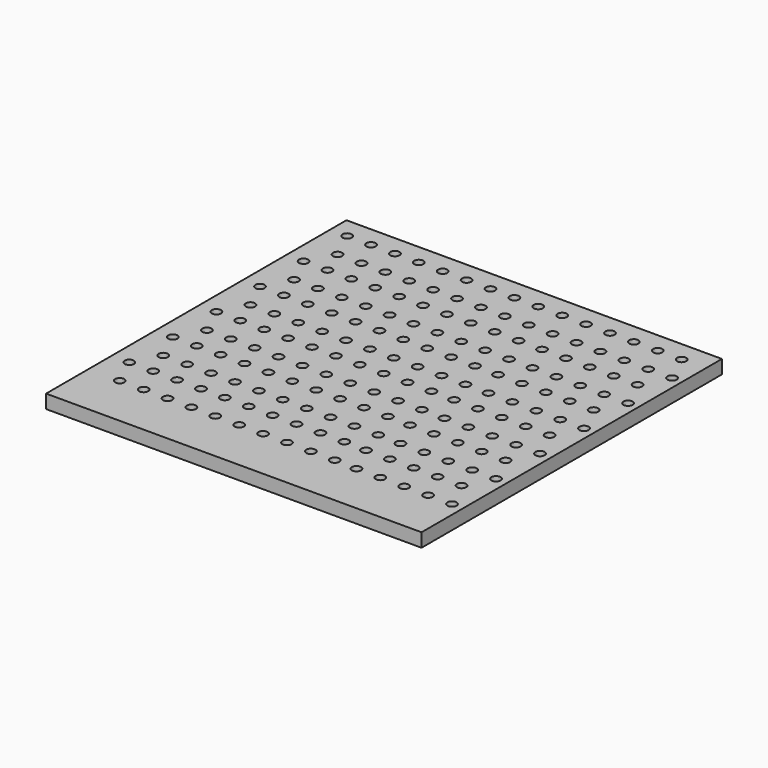
from build123d import *

# Parameters (mm, degrees)
F0_W     = 110
F0_H     = 110
F0_R     = 1.35
F1_DEPTH = 4


# Not quite as in the source:
# - a feature names something its author has since deleted; it is built from what else it names


with BuildPart() as f1:
    # F0 (on Top) → F1 (new body)
    with BuildSketch(Plane.XY):
        with Locations((-18.9387425125, -57.1583950296)):
            Rectangle(F0_W, F0_H)
        with Locations((-64.7594391714, -96.6581940938)):
            Circle(F0_R, mode=Mode.SUBTRACT)
        with Locations((-68.7594391714, -88.1581940938)):
            Circle(F0_R, mode=Mode.SUBTRACT)
        with Locations((-61.7594391714, -88.1581940938)):
            Circle(F0_R, mode=Mode.SUBTRACT)
        with Locations((-57.7594391714, -96.6581940938)):
            Circle(F0_R, mode=Mode.SUBTRACT)
        with Locations((-50.7594391714, -96.6581940938)):
            Circle(F0_R, mode=Mode.SUBTRACT)
        with Locations((-54.7594391714, -88.1581940938)):
            Circle(F0_R, mode=Mode.SUBTRACT)
        with Locations((-47.7594391714, -88.1581940938)):
            Circle(F0_R, mode=Mode.SUBTRACT)
        with Locations((-43.7594391714, -96.6581940938)):
            Circle(F0_R, mode=Mode.SUBTRACT)
        with Locations((-36.7594391714, -96.6581940938)):
            Circle(F0_R, mode=Mode.SUBTRACT)
        with Locations((-40.7594391714, -88.1581940938)):
            Circle(F0_R, mode=Mode.SUBTRACT)
        with Locations((-33.7594391714, -88.1581940938)):
            Circle(F0_R, mode=Mode.SUBTRACT)
        with Locations((-29.7594391714, -96.6581940938)):
            Circle(F0_R, mode=Mode.SUBTRACT)
        with Locations((-22.7594391714, -96.6581940938)):
            Circle(F0_R, mode=Mode.SUBTRACT)
        with Locations((-26.7594391714, -88.1581940938)):
            Circle(F0_R, mode=Mode.SUBTRACT)
        with Locations((-19.7594391714, -88.1581940938)):
            Circle(F0_R, mode=Mode.SUBTRACT)
        with Locations((-64.7952998396, -80.658234281)):
            Circle(F0_R, mode=Mode.SUBTRACT)
        with Locations((-68.7952998396, -72.158234281)):
            Circle(F0_R, mode=Mode.SUBTRACT)
        with Locations((-61.7952998396, -72.158234281)):
            Circle(F0_R, mode=Mode.SUBTRACT)
        with Locations((-57.7952998396, -80.658234281)):
            Circle(F0_R, mode=Mode.SUBTRACT)
        with Locations((-50.7952998396, -80.658234281)):
            Circle(F0_R, mode=Mode.SUBTRACT)
        with Locations((-54.7952998396, -72.158234281)):
            Circle(F0_R, mode=Mode.SUBTRACT)
        with Locations((-47.7952998396, -72.158234281)):
            Circle(F0_R, mode=Mode.SUBTRACT)
        with Locations((-64.8311605078, -64.6582744682)):
            Circle(F0_R, mode=Mode.SUBTRACT)
        with Locations((-57.8311605078, -64.6582744682)):
            Circle(F0_R, mode=Mode.SUBTRACT)
        with Locations((-50.8311605078, -64.6582744682)):
            Circle(F0_R, mode=Mode.SUBTRACT)
        with Locations((-43.7952998396, -80.658234281)):
            Circle(F0_R, mode=Mode.SUBTRACT)
        with Locations((-36.7952998396, -80.658234281)):
            Circle(F0_R, mode=Mode.SUBTRACT)
        with Locations((-40.7952998396, -72.158234281)):
            Circle(F0_R, mode=Mode.SUBTRACT)
        with Locations((-33.7952998396, -72.158234281)):
            Circle(F0_R, mode=Mode.SUBTRACT)
        with Locations((-29.7952998396, -80.658234281)):
            Circle(F0_R, mode=Mode.SUBTRACT)
        with Locations((-22.7952998396, -80.658234281)):
            Circle(F0_R, mode=Mode.SUBTRACT)
        with Locations((-26.7952998396, -72.158234281)):
            Circle(F0_R, mode=Mode.SUBTRACT)
        with Locations((-19.7952998396, -72.158234281)):
            Circle(F0_R, mode=Mode.SUBTRACT)
        with Locations((-43.8311605078, -64.6582744682)):
            Circle(F0_R, mode=Mode.SUBTRACT)
        with Locations((-36.8311605078, -64.6582744682)):
            Circle(F0_R, mode=Mode.SUBTRACT)
        with Locations((-29.8311605078, -64.6582744682)):
            Circle(F0_R, mode=Mode.SUBTRACT)
        with Locations((-22.8311605078, -64.6582744682)):
            Circle(F0_R, mode=Mode.SUBTRACT)
        with Locations((-15.7594391714, -96.6581940938)):
            Circle(F0_R, mode=Mode.SUBTRACT)
        with Locations((-8.7594391714, -96.6581940938)):
            Circle(F0_R, mode=Mode.SUBTRACT)
        with Locations((-12.7594391714, -88.1581940938)):
            Circle(F0_R, mode=Mode.SUBTRACT)
        with Locations((-5.7594391714, -88.1581940938)):
            Circle(F0_R, mode=Mode.SUBTRACT)
        with Locations((-1.7594391714, -96.6581940938)):
            Circle(F0_R, mode=Mode.SUBTRACT)
        with Locations((4.7549700499, -96.8664198815)):
            Circle(F0_R, mode=Mode.SUBTRACT)
        with Locations((0.7549700499, -88.3664198815)):
            Circle(F0_R, mode=Mode.SUBTRACT)
        with Locations((7.7549700499, -88.3664198815)):
            Circle(F0_R, mode=Mode.SUBTRACT)
        with Locations((11.7549700499, -96.8664198815)):
            Circle(F0_R, mode=Mode.SUBTRACT)
        with Locations((18.7549700499, -96.8664198815)):
            Circle(F0_R, mode=Mode.SUBTRACT)
        with Locations((14.7549700499, -88.3664198815)):
            Circle(F0_R, mode=Mode.SUBTRACT)
        with Locations((21.7549700499, -88.3664198815)):
            Circle(F0_R, mode=Mode.SUBTRACT)
        with Locations((25.7549700499, -96.8664198815)):
            Circle(F0_R, mode=Mode.SUBTRACT)
        with Locations((32.7549700499, -96.8664198815)):
            Circle(F0_R, mode=Mode.SUBTRACT)
        with Locations((28.7549700499, -88.3664198815)):
            Circle(F0_R, mode=Mode.SUBTRACT)
        with Locations((-15.7952998396, -80.658234281)):
            Circle(F0_R, mode=Mode.SUBTRACT)
        with Locations((-8.7952998396, -80.658234281)):
            Circle(F0_R, mode=Mode.SUBTRACT)
        with Locations((-12.7952998396, -72.158234281)):
            Circle(F0_R, mode=Mode.SUBTRACT)
        with Locations((-5.7952998396, -72.158234281)):
            Circle(F0_R, mode=Mode.SUBTRACT)
        with Locations((-1.7952998396, -80.658234281)):
            Circle(F0_R, mode=Mode.SUBTRACT)
        with Locations((4.8162275374, -80.8248149111)):
            Circle(F0_R, mode=Mode.SUBTRACT)
        with Locations((0.8162275374, -72.3248149111)):
            Circle(F0_R, mode=Mode.SUBTRACT)
        with Locations((7.8162275374, -72.3248149111)):
            Circle(F0_R, mode=Mode.SUBTRACT)
        with Locations((-15.8311605078, -64.6582744682)):
            Circle(F0_R, mode=Mode.SUBTRACT)
        with Locations((-8.8311605078, -64.6582744682)):
            Circle(F0_R, mode=Mode.SUBTRACT)
        with Locations((-1.8311605078, -64.6582744682)):
            Circle(F0_R, mode=Mode.SUBTRACT)
        with Locations((4.877485025, -64.7832099407)):
            Circle(F0_R, mode=Mode.SUBTRACT)
        with Locations((11.8162275374, -80.8248149111)):
            Circle(F0_R, mode=Mode.SUBTRACT)
        with Locations((18.8162275374, -80.8248149111)):
            Circle(F0_R, mode=Mode.SUBTRACT)
        with Locations((14.8162275374, -72.3248149111)):
            Circle(F0_R, mode=Mode.SUBTRACT)
        with Locations((21.8162275374, -72.3248149111)):
            Circle(F0_R, mode=Mode.SUBTRACT)
        with Locations((25.8162275374, -80.8248149111)):
            Circle(F0_R, mode=Mode.SUBTRACT)
        with Locations((32.8162275374, -80.8248149111)):
            Circle(F0_R, mode=Mode.SUBTRACT)
        with Locations((28.8162275374, -72.3248149111)):
            Circle(F0_R, mode=Mode.SUBTRACT)
        with Locations((11.877485025, -64.7832099407)):
            Circle(F0_R, mode=Mode.SUBTRACT)
        with Locations((18.877485025, -64.7832099407)):
            Circle(F0_R, mode=Mode.SUBTRACT)
        with Locations((25.877485025, -64.7832099407)):
            Circle(F0_R, mode=Mode.SUBTRACT)
        with Locations((32.877485025, -64.7832099407)):
            Circle(F0_R, mode=Mode.SUBTRACT)
        with Locations((-68.8311605078, -56.1582744682)):
            Circle(F0_R, mode=Mode.SUBTRACT)
        with Locations((-61.8311605078, -56.1582744682)):
            Circle(F0_R, mode=Mode.SUBTRACT)
        with Locations((-64.8670211761, -48.6583146553)):
            Circle(F0_R, mode=Mode.SUBTRACT)
        with Locations((-54.8311605078, -56.1582744682)):
            Circle(F0_R, mode=Mode.SUBTRACT)
        with Locations((-47.8311605078, -56.1582744682)):
            Circle(F0_R, mode=Mode.SUBTRACT)
        with Locations((-57.8670211761, -48.6583146553)):
            Circle(F0_R, mode=Mode.SUBTRACT)
        with Locations((-50.8670211761, -48.6583146553)):
            Circle(F0_R, mode=Mode.SUBTRACT)
        with Locations((-68.8670211761, -40.1583146553)):
            Circle(F0_R, mode=Mode.SUBTRACT)
        with Locations((-61.8670211761, -40.1583146553)):
            Circle(F0_R, mode=Mode.SUBTRACT)
        with Locations((-64.9028818443, -32.6583548425)):
            Circle(F0_R, mode=Mode.SUBTRACT)
        with Locations((-54.8670211761, -40.1583146553)):
            Circle(F0_R, mode=Mode.SUBTRACT)
        with Locations((-47.8670211761, -40.1583146553)):
            Circle(F0_R, mode=Mode.SUBTRACT)
        with Locations((-57.9028818443, -32.6583548425)):
            Circle(F0_R, mode=Mode.SUBTRACT)
        with Locations((-50.9028818443, -32.6583548425)):
            Circle(F0_R, mode=Mode.SUBTRACT)
        with Locations((-40.8311605078, -56.1582744682)):
            Circle(F0_R, mode=Mode.SUBTRACT)
        with Locations((-33.8311605078, -56.1582744682)):
            Circle(F0_R, mode=Mode.SUBTRACT)
        with Locations((-43.8670211761, -48.6583146553)):
            Circle(F0_R, mode=Mode.SUBTRACT)
        with Locations((-36.8670211761, -48.6583146553)):
            Circle(F0_R, mode=Mode.SUBTRACT)
        with Locations((-26.8311605078, -56.1582744682)):
            Circle(F0_R, mode=Mode.SUBTRACT)
        with Locations((-19.8311605078, -56.1582744682)):
            Circle(F0_R, mode=Mode.SUBTRACT)
        with Locations((-29.8670211761, -48.6583146553)):
            Circle(F0_R, mode=Mode.SUBTRACT)
        with Locations((-22.8670211761, -48.6583146553)):
            Circle(F0_R, mode=Mode.SUBTRACT)
        with Locations((-40.8670211761, -40.1583146553)):
            Circle(F0_R, mode=Mode.SUBTRACT)
        with Locations((-33.8670211761, -40.1583146553)):
            Circle(F0_R, mode=Mode.SUBTRACT)
        with Locations((-43.9028818443, -32.6583548425)):
            Circle(F0_R, mode=Mode.SUBTRACT)
        with Locations((-36.9028818443, -32.6583548425)):
            Circle(F0_R, mode=Mode.SUBTRACT)
        with Locations((-26.8670211761, -40.1583146553)):
            Circle(F0_R, mode=Mode.SUBTRACT)
        with Locations((-19.8670211761, -40.1583146553)):
            Circle(F0_R, mode=Mode.SUBTRACT)
        with Locations((-29.9028818443, -32.6583548425)):
            Circle(F0_R, mode=Mode.SUBTRACT)
        with Locations((-22.9028818443, -32.6583548425)):
            Circle(F0_R, mode=Mode.SUBTRACT)
        with Locations((-68.9028818443, -24.1583548425)):
            Circle(F0_R, mode=Mode.SUBTRACT)
        with Locations((-61.9028818443, -24.1583548425)):
            Circle(F0_R, mode=Mode.SUBTRACT)
        with Locations((-64.9387425125, -16.6583950296)):
            Circle(F0_R, mode=Mode.SUBTRACT)
        with Locations((-54.9028818443, -24.1583548425)):
            Circle(F0_R, mode=Mode.SUBTRACT)
        with Locations((-47.9028818443, -24.1583548425)):
            Circle(F0_R, mode=Mode.SUBTRACT)
        with Locations((-57.9387425125, -16.6583950296)):
            Circle(F0_R, mode=Mode.SUBTRACT)
        with Locations((-50.9387425125, -16.6583950296)):
            Circle(F0_R, mode=Mode.SUBTRACT)
        with Locations((-68.9387425125, -8.1583950296)):
            Circle(F0_R, mode=Mode.SUBTRACT)
        with Locations((-61.9387425125, -8.1583950296)):
            Circle(F0_R, mode=Mode.SUBTRACT)
        with Locations((-54.9387425125, -8.1583950296)):
            Circle(F0_R, mode=Mode.SUBTRACT)
        with Locations((-47.9387425125, -8.1583950296)):
            Circle(F0_R, mode=Mode.SUBTRACT)
        with Locations((-40.9028818443, -24.1583548425)):
            Circle(F0_R, mode=Mode.SUBTRACT)
        with Locations((-33.9028818443, -24.1583548425)):
            Circle(F0_R, mode=Mode.SUBTRACT)
        with Locations((-43.9387425125, -16.6583950296)):
            Circle(F0_R, mode=Mode.SUBTRACT)
        with Locations((-36.9387425125, -16.6583950296)):
            Circle(F0_R, mode=Mode.SUBTRACT)
        with Locations((-26.9028818443, -24.1583548425)):
            Circle(F0_R, mode=Mode.SUBTRACT)
        with Locations((-19.9028818443, -24.1583548425)):
            Circle(F0_R, mode=Mode.SUBTRACT)
        with Locations((-29.9387425125, -16.6583950296)):
            Circle(F0_R, mode=Mode.SUBTRACT)
        with Locations((-22.9387425125, -16.6583950296)):
            Circle(F0_R, mode=Mode.SUBTRACT)
        with Locations((-40.9387425125, -8.1583950296)):
            Circle(F0_R, mode=Mode.SUBTRACT)
        with Locations((-33.9387425125, -8.1583950296)):
            Circle(F0_R, mode=Mode.SUBTRACT)
        with Locations((-26.9387425125, -8.1583950296)):
            Circle(F0_R, mode=Mode.SUBTRACT)
        with Locations((-19.9387425125, -8.1583950296)):
            Circle(F0_R, mode=Mode.SUBTRACT)
        with Locations((-12.8311605078, -56.1582744682)):
            Circle(F0_R, mode=Mode.SUBTRACT)
        with Locations((-5.8311605078, -56.1582744682)):
            Circle(F0_R, mode=Mode.SUBTRACT)
        with Locations((-15.8670211761, -48.6583146553)):
            Circle(F0_R, mode=Mode.SUBTRACT)
        with Locations((-8.8670211761, -48.6583146553)):
            Circle(F0_R, mode=Mode.SUBTRACT)
        with Locations((0.877485025, -56.2832099407)):
            Circle(F0_R, mode=Mode.SUBTRACT)
        with Locations((7.877485025, -56.2832099407)):
            Circle(F0_R, mode=Mode.SUBTRACT)
        with Locations((-1.8670211761, -48.6583146553)):
            Circle(F0_R, mode=Mode.SUBTRACT)
        with Locations((4.9387425125, -48.7416049704)):
            Circle(F0_R, mode=Mode.SUBTRACT)
        with Locations((-12.8670211761, -40.1583146553)):
            Circle(F0_R, mode=Mode.SUBTRACT)
        with Locations((-5.8670211761, -40.1583146553)):
            Circle(F0_R, mode=Mode.SUBTRACT)
        with Locations((-15.9028818443, -32.6583548425)):
            Circle(F0_R, mode=Mode.SUBTRACT)
        with Locations((-8.9028818443, -32.6583548425)):
            Circle(F0_R, mode=Mode.SUBTRACT)
        with Locations((0.9387425125, -40.2416049704)):
            Circle(F0_R, mode=Mode.SUBTRACT)
        with Locations((7.9387425125, -40.2416049704)):
            Circle(F0_R, mode=Mode.SUBTRACT)
        with Locations((-1.9028818443, -32.6583548425)):
            Circle(F0_R, mode=Mode.SUBTRACT)
        with Locations((5, -32.7)):
            Circle(F0_R, mode=Mode.SUBTRACT)
        with Locations((14.877485025, -56.2832099407)):
            Circle(F0_R, mode=Mode.SUBTRACT)
        with Locations((21.877485025, -56.2832099407)):
            Circle(F0_R, mode=Mode.SUBTRACT)
        with Locations((11.9387425125, -48.7416049704)):
            Circle(F0_R, mode=Mode.SUBTRACT)
        with Locations((18.9387425125, -48.7416049704)):
            Circle(F0_R, mode=Mode.SUBTRACT)
        with Locations((28.877485025, -56.2832099407)):
            Circle(F0_R, mode=Mode.SUBTRACT)
        with Locations((25.9387425125, -48.7416049704)):
            Circle(F0_R, mode=Mode.SUBTRACT)
        with Locations((32.9387425125, -48.7416049704)):
            Circle(F0_R, mode=Mode.SUBTRACT)
        with Locations((14.9387425125, -40.2416049704)):
            Circle(F0_R, mode=Mode.SUBTRACT)
        with Locations((21.9387425125, -40.2416049704)):
            Circle(F0_R, mode=Mode.SUBTRACT)
        with Locations((12, -32.7)):
            Circle(F0_R, mode=Mode.SUBTRACT)
        with Locations((19, -32.7)):
            Circle(F0_R, mode=Mode.SUBTRACT)
        with Locations((28.9387425125, -40.2416049704)):
            Circle(F0_R, mode=Mode.SUBTRACT)
        with Locations((26, -32.7)):
            Circle(F0_R, mode=Mode.SUBTRACT)
        with Locations((33, -32.7)):
            Circle(F0_R, mode=Mode.SUBTRACT)
        with Locations((-12.9028818443, -24.1583548425)):
            Circle(F0_R, mode=Mode.SUBTRACT)
        with Locations((-5.9028818443, -24.1583548425)):
            Circle(F0_R, mode=Mode.SUBTRACT)
        with Locations((-15.9387425125, -16.6583950296)):
            Circle(F0_R, mode=Mode.SUBTRACT)
        with Locations((-8.9387425125, -16.6583950296)):
            Circle(F0_R, mode=Mode.SUBTRACT)
        with Locations((1, -24.2)):
            Circle(F0_R, mode=Mode.SUBTRACT)
        with Locations((8, -24.2)):
            Circle(F0_R, mode=Mode.SUBTRACT)
        with Locations((-1.9387425125, -16.6583950296)):
            Circle(F0_R, mode=Mode.SUBTRACT)
        with Locations((5.0612574875, -16.6583950296)):
            Circle(F0_R, mode=Mode.SUBTRACT)
        with Locations((-12.9387425125, -8.1583950296)):
            Circle(F0_R, mode=Mode.SUBTRACT)
        with Locations((-5.9387425125, -8.1583950296)):
            Circle(F0_R, mode=Mode.SUBTRACT)
        with Locations((1.0612574875, -8.1583950296)):
            Circle(F0_R, mode=Mode.SUBTRACT)
        with Locations((8.0612574875, -8.1583950296)):
            Circle(F0_R, mode=Mode.SUBTRACT)
        with Locations((15, -24.2)):
            Circle(F0_R, mode=Mode.SUBTRACT)
        with Locations((22, -24.2)):
            Circle(F0_R, mode=Mode.SUBTRACT)
        with Locations((12.0612574875, -16.6583950296)):
            Circle(F0_R, mode=Mode.SUBTRACT)
        with Locations((19.0612574875, -16.6583950296)):
            Circle(F0_R, mode=Mode.SUBTRACT)
        with Locations((29, -24.2)):
            Circle(F0_R, mode=Mode.SUBTRACT)
        with Locations((26.0612574875, -16.6583950296)):
            Circle(F0_R, mode=Mode.SUBTRACT)
        with Locations((33.0612574875, -16.6583950296)):
            Circle(F0_R, mode=Mode.SUBTRACT)
        with Locations((15.0612574875, -8.1583950296)):
            Circle(F0_R, mode=Mode.SUBTRACT)
        with Locations((22.0612574875, -8.1583950296)):
            Circle(F0_R, mode=Mode.SUBTRACT)
        with Locations((29.0612574875, -8.1583950296)):
            Circle(F0_R, mode=Mode.SUBTRACT)
    extrude(amount=F1_DEPTH)


solid = f1.part
